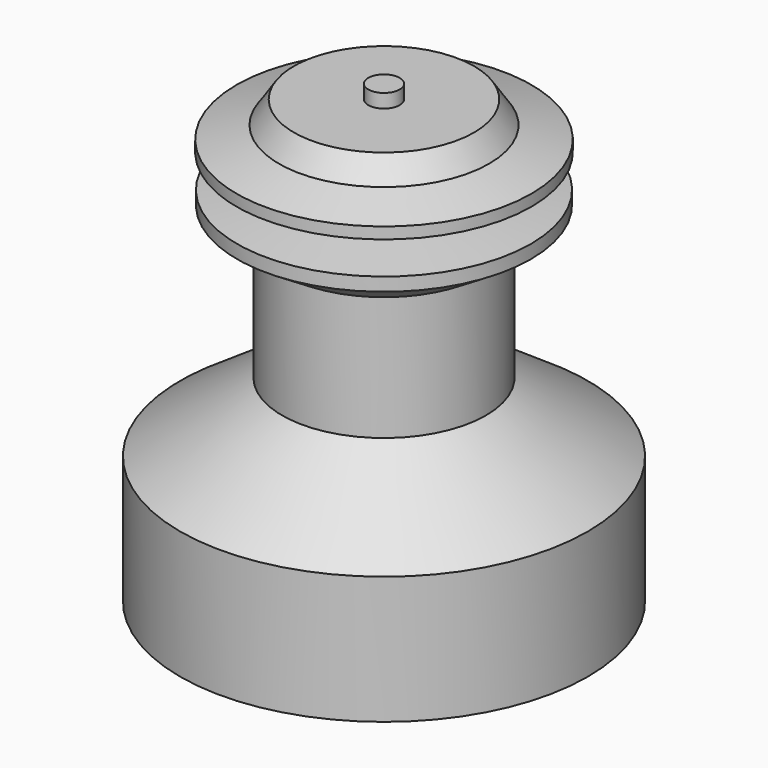
from build123d import *


# Not quite as in the source:
# - the program builds the solid bodies; features that only make, move or delete a surface that nothing else refers to are left out


with BuildPart() as f1:
    # F0 (on Front) → F1 (revolve)
    with BuildSketch(Plane.XZ):
        Polygon((242.856904766, 297), (234, 297), (234, 40), (349, 40), (349, 112.0852836363), (291.5, 151), (291.5, 220.900633561), (316.8506103335, 236.8069001733), (316.8506103335, 244.3618179582), (284.5458486148, 248.6925777132), (284.5458486148, 257.150895566), (317.1651528727, 262.9498915393), (317.1651528727, 269.3958750746), (293.2726186624, 276.5128102049), (284.7837560136, 289.2461182581), (242.856904766, 289.2461182581), align=None)
    revolve(axis=Axis((234, 0, 171.6133333333), (0, 0, -1)))


solid = f1.part
